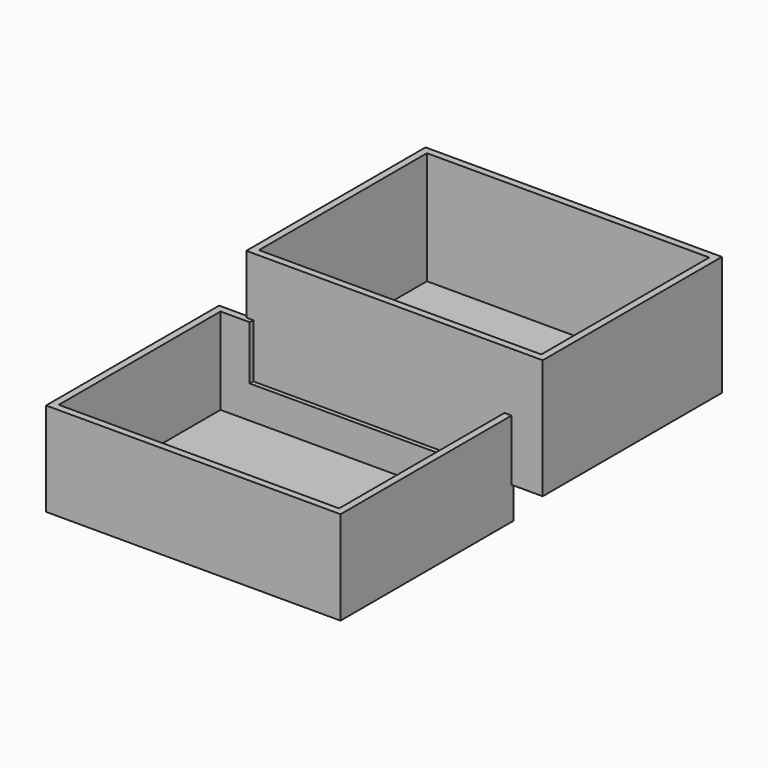
from build123d import *

# Parameters (mm, degrees)
F0_W     = 106.8777292967
F0_H     = 43.1794375181
F1_DEPTH = 80.772
F2_T     = -2.54
F3_W     = 106.1705686152
F3_H     = 77.9809653759
F4_DEPTH = 33.782
F5_T     = -2.54


# Not quite as in the source:
# - a shell that OpenCascade refuses in one call is made with other operations: the cavity is built on its own and cut out


with BuildPart() as f1:
    # F0 (on Front) → F1 (new body)
    with BuildSketch(Plane.XZ):
        with Locations((-4.4315196574, 33.3908237517)):
            Rectangle(F0_W, F0_H)
    extrude(amount=F1_DEPTH)

    # F2
    f2_openings = [f1.faces().sort_by_distance(p)[0] for p in [
        (-4.43152, -40.386, 54.980543),
    ]]
    offset(amount=F2_T, openings=f2_openings)

    # F3 (on Top) → F4 (join)
    with BuildSketch(Plane.XY):
        with Locations((-15.3196584433, -118.8506782055)):
            Rectangle(F3_W, F3_H)
    extrude(amount=F4_DEPTH)

    # F5: a shell. OpenCascade refuses it in one call, so the cavity is built on its own and cut out:
    # the body offset inwards by the wall thickness, plus a prism from it out through each open face.
    f5_core = offset(f1.part, amount=F5_T, kind=Kind.INTERSECTION, mode=Mode.PRIVATE)
    f5_exits = [f5_core.faces().sort_by_distance(p)[0] for p in [
        (-15.216343, -118.119753, 31.242),
    ]]
    add(f5_core, mode=Mode.SUBTRACT)
    extrude(f5_exits, amount=-F5_T, mode=Mode.SUBTRACT)


solid = f1.part
